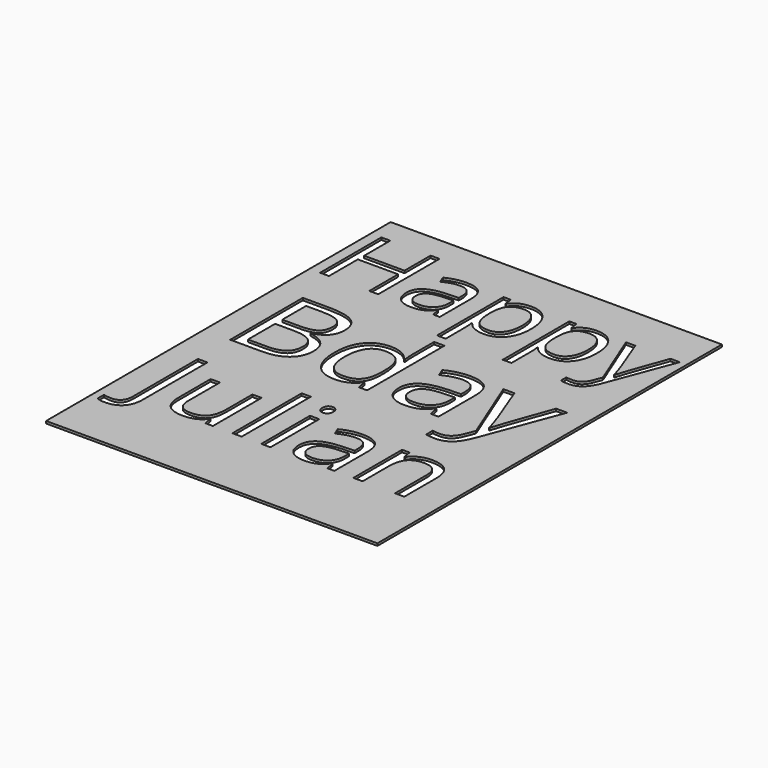
from build123d import *

# Parameters (mm, degrees)
F0_W         = 100
F0_H         = 130
F1_DEPTH     = 0.7
F2_TEXT_SIZE = 32.390303153
F5_DEPTH     = 0.701
F3_TEXT_SIZE = 38.387669633
F6_DEPTH     = 0.7010001
F4_TEXT_SIZE = 34.3634411168
F7_DEPTH     = 0.7010001


# Not quite as in the source:
# - Text() gives the source's letters only with a copy of the font that has no kerning and outlines rounded to 1/6400 em; it was checked with that copy


with BuildPart() as f1:
    # F0 (on Top) → F1 (new body)
    with BuildSketch(Plane.XY):
        Rectangle(F0_W, F0_H)
    extrude(amount=F1_DEPTH)

    # F2 (on face) → F5 (cut, through all)
    with BuildSketch(Plane.XY.offset(0.7)):
        with Locations((-50, 34.4092040184)):
            Text('Happy', F2_TEXT_SIZE, font='Open Sans', text_align=(TextAlign.LEFT, TextAlign.BOTTOM))
    extrude(amount=-F5_DEPTH, mode=Mode.SUBTRACT)

    # F3 (on face) → F6 (cut, through all)
    with BuildSketch(Plane.XY.offset(0.7)):
        with Locations((-45.771297964, -5.5289105512)):
            Text('Bday', F3_TEXT_SIZE, font='Open Sans', text_align=(TextAlign.LEFT, TextAlign.BOTTOM))
    extrude(amount=-F6_DEPTH, mode=Mode.SUBTRACT)

    # F4 (on face) → F7 (cut, through all)
    with BuildSketch(Plane.XY.offset(0.7)):
        with Locations((-45, -42.458436705)):
            Text('Julian', F4_TEXT_SIZE, font='Open Sans', text_align=(TextAlign.LEFT, TextAlign.BOTTOM))
    extrude(amount=-F7_DEPTH, mode=Mode.SUBTRACT)


solid = f1.part
